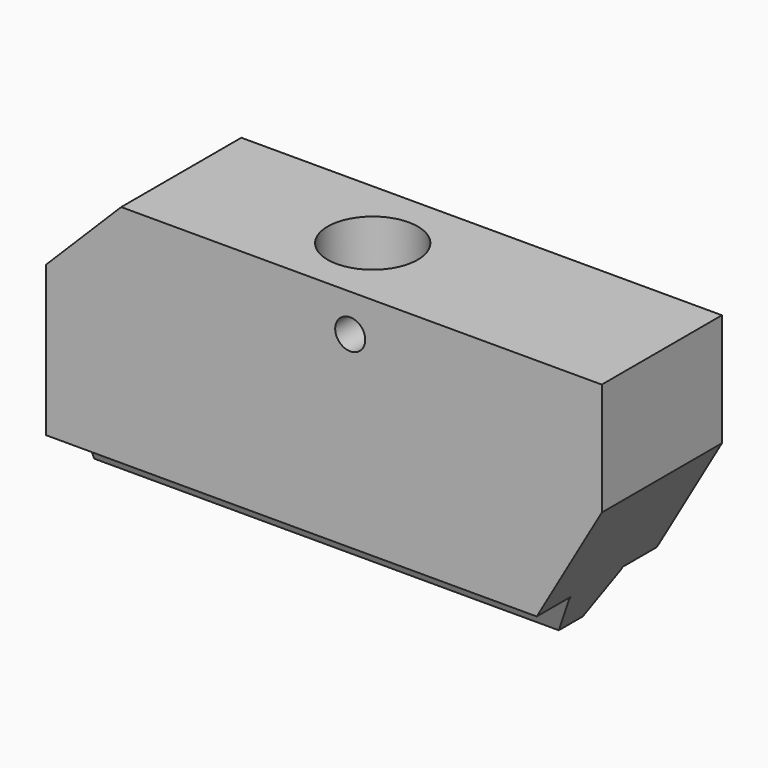
from build123d import *

# Parameters (mm, degrees)
F1_DEPTH     = 11.5
F3_DEPTH     = 5
F5_D         = 14
F5_DEPTH     = 36
F5_TIP       = 4.2060243332
F7_D         = 6.8
F7_DEPTH     = 17
F7_TIP       = 2.0429261047
F8_SIZE2     = 9.237604307
F8_SIZE      = 16
F8_2_SIZE2   = 9.237604307
F8_2_SIZE    = 16
F9_T1_DEPTH  = 23
F9_T6_DEPTH  = 84.5247913859
F9_T12_DEPTH = 98.4752086141
F9_T18_DEPTH = 98.4752086141
F9_T25_DEPTH = 98.4752086141
F9_T32_DEPTH = 98.4752086141
F9_T38_DEPTH = 98.4752086141
F9_T44_DEPTH = 98.4752086141
F9_T51_DEPTH = 98.4752086141
F9_T58_DEPTH = 98.4752086141
F11_DEPTH    = 74
F13_DEPTH    = 20
F14_SIZE2    = 10
F14_SIZE     = 10
F16_D        = 12
F16_DEPTH    = 12
F16_TIP      = 3.6051637142
F17_R        = 2
F18_DEPTH    = 20
F21_D        = 6
F21_DEPTH    = 8
F21_TIP      = 1.8025818571


# Not quite as in the source:
# - a fillet or chamfer that OpenCascade refuses, or shapes differently, is made with other operations: its cross-section is extruded or revolved along the edge and cut away or added


with BuildPart() as f1:
    # F0 (on Front) → F1 (new body, symmetric)
    with BuildSketch(Plane.XZ):
        Polygon((-200, 0), (0, 0), (0, 40), (-63, 40), (-63, 155), (0, 155), (0, 185), (-90, 185), (-200, 30), align=None)
    extrude(amount=F1_DEPTH, both=True)

    # F2 (on face) → F3 (cut)
    with BuildSketch(Plane.YZ.offset(-63)):
        with BuildLine():
            ThreePointArc((3.5, 135), (0, 138.5), (-3.5, 135))
            Line((-3.5, 135), (-3.5, 67))
            ThreePointArc((-3.5, 67), (0, 63.5), (3.5, 67))
            Line((3.5, 67), (3.5, 135))
        make_face()
    extrude(amount=-F3_DEPTH, mode=Mode.SUBTRACT)

    # F5
    with Locations(Plane.XY.offset(185)):
        with Locations((-20, 0)):
            Hole(F5_D / 2, depth=F5_DEPTH)
            with Locations((0, 0, -(F5_DEPTH + F5_TIP / 2))):  # 118° drill point
                Cone(0, F5_D / 2, F5_TIP, mode=Mode.SUBTRACT)

    # F7
    with Locations(Plane(origin=(0, 0, 0), x_dir=(1, 0, 0), z_dir=(0, 0, -1))):
        with Locations((-175, 0), (-125, 0), (-75, 0), (-25, 0)):
            Hole(F7_D / 2, depth=F7_DEPTH)
            with Locations((0, 0, -(F7_DEPTH + F7_TIP / 2))):  # 118° drill point
                Cone(0, F7_D / 2, F7_TIP, mode=Mode.SUBTRACT)

    # F8
    f8_edges = [f1.edges().sort_by_distance(p)[0] for p in [
        (-31.5, -11.5, 40),
    ]]
    f8_side = f1.faces().sort_by_distance((-97.944693, -11.5, 74.396883))[0]
    chamfer(f8_edges, length=F8_SIZE, length2=F8_SIZE2, reference=f8_side)

    # F8#2
    f8_2_edges = [f1.edges().sort_by_distance(p)[0] for p in [
        (-31.5, 11.5, 40),
    ]]
    f8_2_side = f1.faces().sort_by_distance((-97.944693, 11.5, 74.396883))[0]
    chamfer(f8_2_edges, length=F8_2_SIZE, length2=F8_2_SIZE2, reference=f8_2_side)

    # F9: fillet of radius 16 on 4 edges, made by hand

    # F9_s2 → F9_t1 (join)
    with BuildSketch(Plane.XZ.offset(-11.5)):
        with BuildLine():
            ThreePointArc((-63, 139), (-58.313708499, 150.313708499), (-47, 155))
            Line((-47, 155), (-63, 155))
            Line((-63, 155), (-63, 139))
        make_face()
    extrude(amount=F9_T1_DEPTH)


with BuildPart() as f9_tool4:
    # F9_s5 → F9_t6 (new body)
    with BuildSketch(Plane.XZ.offset(-42.262395693)):
        with BuildLine():
            ThreePointArc((-47, 40), (-58.313708499, 44.686291501), (-63, 56))
            Line((-63, 56), (-63, 40))
            Line((-63, 40), (-47, 40))
        make_face()
    extrude(amount=F9_T6_DEPTH)

    split(bisect_by=Plane.XZ.offset(-11.5), keep=Keep.TOP)

    split(bisect_by=Plane.XZ.offset(11.5), keep=Keep.BOTTOM)


with BuildPart() as f1_1:
    add(f1.part)

    # F9_t3: union F9_tool4
    add(f9_tool4.part)


with BuildPart() as f9_tool10:
    # F9_s11 → F9_t12 (new body)
    with BuildSketch(Plane(origin=(0, -12.4826951546, -21.6206622231), x_dir=(1, 0, 0), z_dir=(0, 0.5, 0.8660254038))):
        with BuildLine():
            ThreePointArc((-47, -21.9592921435), (-58.313708499, -26.6455836445), (-63, -37.9592921435))
            Line((-63, -37.9592921435), (-63, -21.9592921435))
            Line((-63, -21.9592921435), (-47, -21.9592921435))
        make_face()
    extrude(amount=F9_T12_DEPTH)

    split(bisect_by=Plane.XY.offset(40), keep=Keep.BOTTOM)

    split(bisect_by=Plane.XZ.offset(11.5), keep=Keep.TOP)


with BuildPart() as f1_2:
    add(f1_1.part)

    # F9_t9: union F9_tool10
    add(f9_tool10.part)


with BuildPart() as f9_tool16:
    # F9_s17 → F9_t18 (new body)
    with BuildSketch(Plane(origin=(0, -12.4826951546, -21.6206622231), x_dir=(1, 0, 0), z_dir=(0, 0.5, 0.8660254038))):
        with BuildLine():
            ThreePointArc((-47, -21.9592921435), (-58.313708499, -26.6455836445), (-63, -37.9592921435))
            Line((-63, -37.9592921435), (-63, -21.9592921435))
            Line((-63, -21.9592921435), (-47, -21.9592921435))
        make_face()
    extrude(amount=F9_T18_DEPTH)

    split(bisect_by=Plane.XY.offset(40), keep=Keep.BOTTOM)

    split(bisect_by=Plane.XZ.offset(11.5), keep=Keep.BOTTOM)

    split(bisect_by=Plane.XZ.offset(3.5), keep=Keep.TOP)


with BuildPart() as f1_3:
    add(f1_2.part)

    # F9_t15: union F9_tool16
    add(f9_tool16.part)


with BuildPart() as f9_tool23:
    # F9_s24 → F9_t25 (new body)
    with BuildSketch(Plane(origin=(0, -12.4826951546, -21.6206622231), x_dir=(1, 0, 0), z_dir=(0, 0.5, 0.8660254038))):
        with BuildLine():
            ThreePointArc((-47, -21.9592921435), (-58.313708499, -26.6455836445), (-63, -37.9592921435))
            Line((-63, -37.9592921435), (-63, -21.9592921435))
            Line((-63, -21.9592921435), (-47, -21.9592921435))
        make_face()
    extrude(amount=F9_T25_DEPTH)

    split(bisect_by=Plane.XY.offset(40), keep=Keep.TOP)

    split(bisect_by=Plane.XZ.offset(11.5), keep=Keep.BOTTOM)

    split(bisect_by=Plane.XZ.offset(3.5), keep=Keep.TOP)


with BuildPart() as f1_4:
    add(f1_3.part)

    # F9_t22: union F9_tool23
    add(f9_tool23.part)


with BuildPart() as f9_tool30:
    # F9_s31 → F9_t32 (new body)
    with BuildSketch(Plane(origin=(0, -12.4826951546, -21.6206622231), x_dir=(1, 0, 0), z_dir=(0, 0.5, 0.8660254038))):
        with BuildLine():
            ThreePointArc((-47, -21.9592921435), (-58.313708499, -26.6455836445), (-63, -37.9592921435))
            Line((-63, -37.9592921435), (-63, -21.9592921435))
            Line((-63, -21.9592921435), (-47, -21.9592921435))
        make_face()
    extrude(amount=F9_T32_DEPTH)

    split(bisect_by=Plane.XY.offset(40), keep=Keep.BOTTOM)

    split(bisect_by=Plane.XZ.offset(3.5), keep=Keep.BOTTOM)


with BuildPart() as f1_5:
    add(f1_4.part)

    # F9_t29: union F9_tool30
    add(f9_tool30.part)


with BuildPart() as f9_tool36:
    # F9_s37 → F9_t38 (new body)
    with BuildSketch(Plane(origin=(0, 12.4826951546, -21.6206622231), x_dir=(1, 0, 0), z_dir=(0, -0.5, 0.8660254038))):
        with BuildLine():
            ThreePointArc((-47, 21.9592921435), (-58.313708499, 26.6455836445), (-63, 37.9592921435))
            Line((-63, 37.9592921435), (-63, 21.9592921435))
            Line((-63, 21.9592921435), (-47, 21.9592921435))
        make_face()
    extrude(amount=F9_T38_DEPTH)

    split(bisect_by=Plane.XY.offset(40), keep=Keep.BOTTOM)

    split(bisect_by=Plane.XZ.offset(-11.5), keep=Keep.BOTTOM)


with BuildPart() as f1_6:
    add(f1_5.part)

    # F9_t35: union F9_tool36
    add(f9_tool36.part)


with BuildPart() as f9_tool42:
    # F9_s43 → F9_t44 (new body)
    with BuildSketch(Plane(origin=(0, 12.4826951546, -21.6206622231), x_dir=(1, 0, 0), z_dir=(0, -0.5, 0.8660254038))):
        with BuildLine():
            ThreePointArc((-47, 21.9592921435), (-58.313708499, 26.6455836445), (-63, 37.9592921435))
            Line((-63, 37.9592921435), (-63, 21.9592921435))
            Line((-63, 21.9592921435), (-47, 21.9592921435))
        make_face()
    extrude(amount=F9_T44_DEPTH)

    split(bisect_by=Plane.XY.offset(40), keep=Keep.BOTTOM)

    split(bisect_by=Plane.XZ.offset(-11.5), keep=Keep.TOP)

    split(bisect_by=Plane.XZ.offset(-3.5), keep=Keep.BOTTOM)


with BuildPart() as f1_7:
    add(f1_6.part)

    # F9_t41: union F9_tool42
    add(f9_tool42.part)


with BuildPart() as f9_tool49:
    # F9_s50 → F9_t51 (new body)
    with BuildSketch(Plane(origin=(0, 12.4826951546, -21.6206622231), x_dir=(1, 0, 0), z_dir=(0, -0.5, 0.8660254038))):
        with BuildLine():
            ThreePointArc((-47, 21.9592921435), (-58.313708499, 26.6455836445), (-63, 37.9592921435))
            Line((-63, 37.9592921435), (-63, 21.9592921435))
            Line((-63, 21.9592921435), (-47, 21.9592921435))
        make_face()
    extrude(amount=F9_T51_DEPTH)

    split(bisect_by=Plane.XY.offset(40), keep=Keep.TOP)

    split(bisect_by=Plane.XZ.offset(-11.5), keep=Keep.TOP)

    split(bisect_by=Plane.XZ.offset(-3.5), keep=Keep.BOTTOM)


with BuildPart() as f1_8:
    add(f1_7.part)

    # F9_t48: union F9_tool49
    add(f9_tool49.part)


with BuildPart() as f9_tool56:
    # F9_s57 → F9_t58 (new body)
    with BuildSketch(Plane(origin=(0, 12.4826951546, -21.6206622231), x_dir=(1, 0, 0), z_dir=(0, -0.5, 0.8660254038))):
        with BuildLine():
            ThreePointArc((-47, 21.9592921435), (-58.313708499, 26.6455836445), (-63, 37.9592921435))
            Line((-63, 37.9592921435), (-63, 21.9592921435))
            Line((-63, 21.9592921435), (-47, 21.9592921435))
        make_face()
    extrude(amount=F9_T58_DEPTH)

    split(bisect_by=Plane.XY.offset(40), keep=Keep.BOTTOM)

    split(bisect_by=Plane.XZ.offset(-3.5), keep=Keep.TOP)


with BuildPart() as f1_9:
    add(f1_8.part)

    # F9_t55: union F9_tool56
    add(f9_tool56.part)


with BuildPart() as f11:
    # F10 (on Right) → F11 (new body)
    with BuildSketch(Plane.YZ):
        Polygon((-2, 90), (0, 90), (2, 90), (4.3, 95.5526911935), (4.3, 96), (10, 96), (10, 126), (0, 126), (-10, 126), (-10, 96), (-4.3, 96), (-4.3, 95.5526911935), align=None)
    extrude(amount=-F11_DEPTH)

    # F12 (on face) → F13 (cut, through all)
    with BuildSketch(Plane.XZ.offset(10)):
        Polygon((0, 90), (0, 111), (-12.124355653, 90), align=None)
    extrude(amount=-F13_DEPTH, mode=Mode.SUBTRACT)

    # F14
    f14_edges = [f11.edges().sort_by_distance(p)[0] for p in [
        (-74, 0, 126),
    ]]
    chamfer(f14_edges, length=F14_SIZE, length2=F14_SIZE2)

    # F16
    with Locations(Plane.XY.offset(126)):
        with Locations((-38.5, 0)):
            Hole(F16_D / 2, depth=F16_DEPTH)
            with Locations((0, 0, -(F16_DEPTH + F16_TIP / 2))):  # 118° drill point
                Cone(0, F16_D / 2, F16_TIP, mode=Mode.SUBTRACT)

    # F17 (on face) → F18 (cut, through all)
    with BuildSketch(Plane.XZ.offset(10)):
        with Locations((-33.5, 121)):
            Circle(F17_R)
    extrude(amount=-F18_DEPTH, mode=Mode.SUBTRACT)

    # F21
    with Locations(Plane(origin=(-74, 0, 0), x_dir=(0, -1, 0), z_dir=(-1, 0, 0))):
        with Locations((0, 108)):
            Hole(F21_D / 2, depth=F21_DEPTH)
            with Locations((0, 0, -(F21_DEPTH + F21_TIP / 2))):  # 118° drill point
                Cone(0, F21_D / 2, F21_TIP, mode=Mode.SUBTRACT)


solid = f11.part
